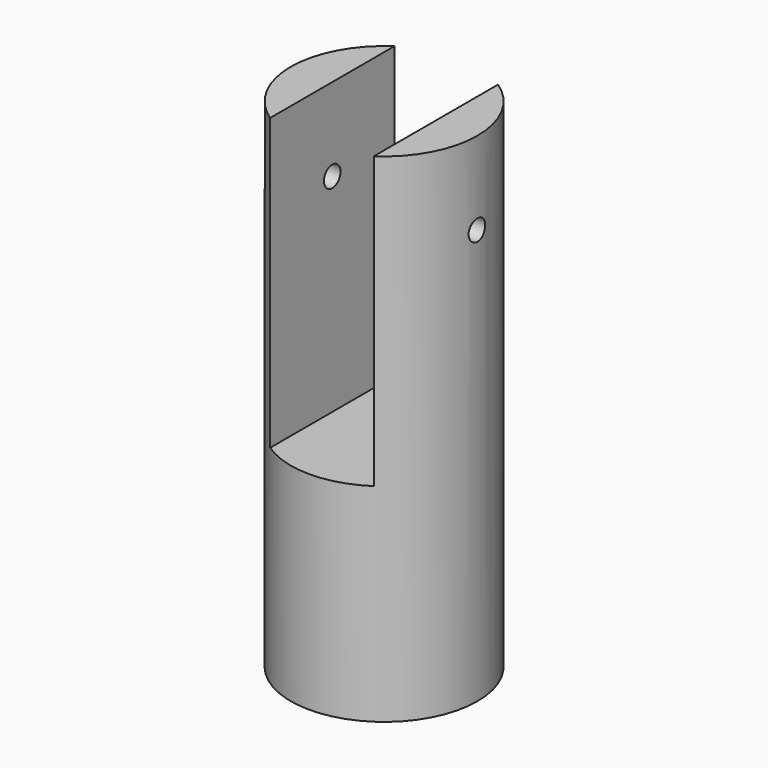
from build123d import *

# Parameters (mm, degrees)
F0_R     = 22.5
F1_DEPTH = 120
F3_DEPTH = 70
F4_R     = 20
F5_DEPTH = 35
F8_D     = 5


# Not quite as in the source:
# - a feature names something its author has since deleted; it is built from what else it names


with BuildPart() as f1:
    # F0 (on Top) → F1 (new body)
    with BuildSketch(Plane.XY):
        Circle(F0_R)
    extrude(amount=F1_DEPTH)

    # F2 (on face) → F3 (cut)
    with BuildSketch(Plane.XY.offset(120)):
        with BuildLine():
            ThreePointArc((12.5, 18.7082869339), (0, 22.5), (-12.5, 18.7082869339))
            Line((-12.5, 18.7082869339), (-12.5, -18.7082869339))
            ThreePointArc((-12.5, -18.7082869339), (0, -22.5), (12.5, -18.7082869339))
            Line((12.5, -18.7082869339), (12.5, 18.7082869339))
        make_face()
    extrude(amount=-F3_DEPTH, mode=Mode.SUBTRACT)

    # F4 (on face) → F5 (cut)
    with BuildSketch(Plane(origin=(0, 0, 0), x_dir=(1, 0, 0), z_dir=(0, 0, -1))):
        Circle(F4_R)
    extrude(amount=-F5_DEPTH, mode=Mode.SUBTRACT)

    # F8 (through all)
    with Locations(Plane.YZ.offset(22.5)):
        with Locations((0, 100)):
            Hole(F8_D / 2)


solid = f1.part
